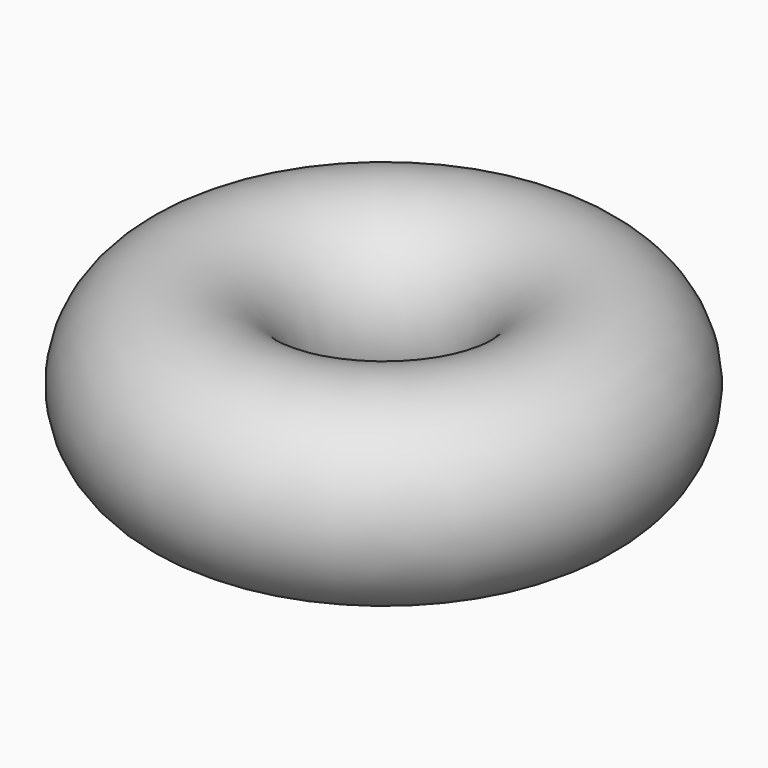
from build123d import *

# Parameters (mm, degrees)
F0_R = 12.7


# Not quite as in the source:
# - a feature of the source that left no trace in its solid (it failed there, or was rolled back) is left out


with BuildPart() as f1:
    # F0 (on Front) → F1 (revolve)
    with BuildSketch(Plane.XZ):
        Circle(F0_R)
    revolve(axis=Axis((22.421406582, 0, 12.001499068), (0, 0, 1)))


solid = f1.part
